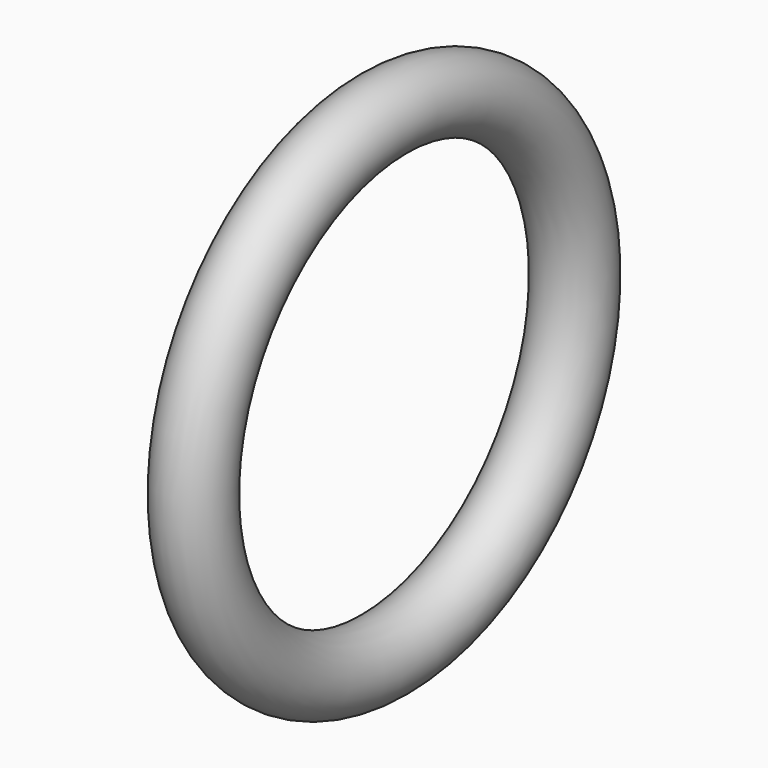
from build123d import *

# Parameters (mm, degrees)
F0_R = 1.5


# Not quite as in the source:
# - the program builds the solid bodies; features that only make, move or delete a surface that nothing else refers to are left out


with BuildPart() as f1:
    # F0 (on Front) → F1 (revolve)
    with BuildSketch(Plane.XZ):
        with Locations((0, 10)):
            Circle(F0_R)
    revolve(axis=Axis((5, 0, 0), (1, 0, 0)))


solid = f1.part
